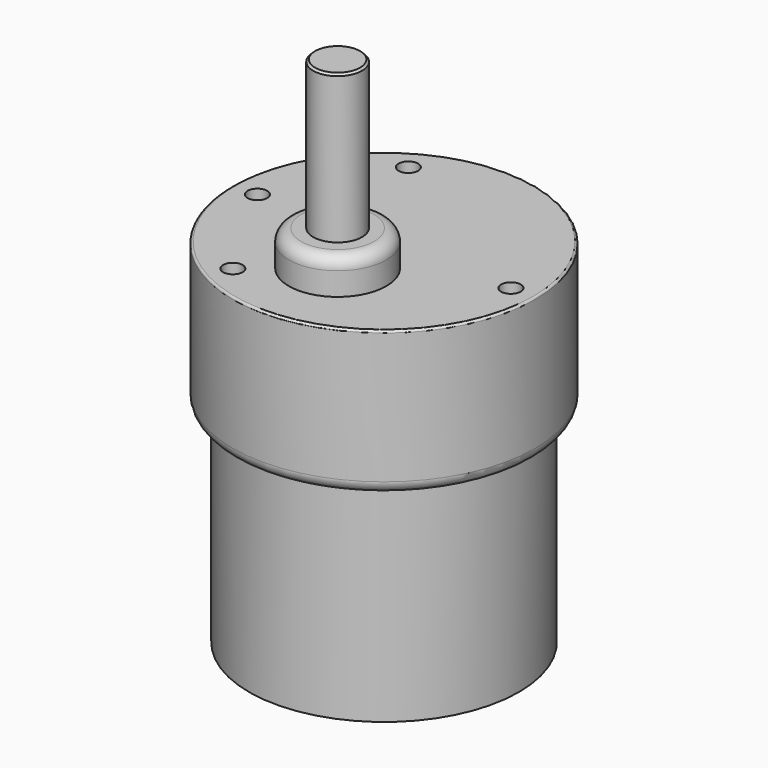
from build123d import *

# Parameters (mm, degrees)
F0_R         = 18.5
F0_R_2       = 16.51
F1_DEPTH     = 17.78
F2_R         = 5.969
F3_DEPTH     = 4.318
F4_R         = 3
F5_DEPTH     = 18.161
F7_DEPTH     = 12
F8_DEPTH     = 25.4
F9_R         = 4.445
F10_DEPTH    = 2.54
F11_R        = 0.635
F12_R        = 1.5
F13_R        = 1.5
F14_R        = 0.25
F15_T2_ANGLE = 276.1399558047
F15_T4_ANGLE = 96.0574088809
F16_D        = 2.4
F16_DEPTH    = 5
F16_TIP      = 0.7210327428


# Not quite as in the source:
# - a fillet or chamfer that OpenCascade refuses, or shapes differently, is made with other operations: its cross-section is extruded or revolved along the edge and cut away or added


with BuildPart() as f1:
    # F0 (on Top) → F1 (new body)
    with BuildSketch(Plane.XY):
        Circle(F0_R)
        Circle(F0_R_2, mode=Mode.SUBTRACT)
        Circle(F0_R_2)
    extrude(amount=F1_DEPTH)

    # F2 (on face) → F3 (join)
    with BuildSketch(Plane.XY.offset(17.78)):
        with Locations((0, -7.0954)):
            Circle(F2_R)
    extrude(amount=F3_DEPTH)

    # F0 (on Top) → F8 (join)
    with BuildSketch(Plane.XY):
        Circle(F0_R_2)
    extrude(amount=-F8_DEPTH)

    # F9 (on face) → F10 (join)
    with BuildSketch(Plane(origin=(0, 0, -25.4), x_dir=(1, 0, 0), z_dir=(0, 0, -1))):
        Circle(F9_R)
    extrude(amount=F10_DEPTH)

    # F11
    f11_edges = [f1.edges().sort_by_distance(p)[0] for p in [
        (-4.445, 0, -27.94),
    ]]
    fillet(f11_edges, radius=F11_R)

    # F12
    f12_edges = [f1.edges().sort_by_distance(p)[0] for p in [
        (-18.5, 0, 0),
    ]]
    fillet(f12_edges, radius=F12_R)

    # F13
    f13_edges = [f1.edges().sort_by_distance(p)[0] for p in [
        (-5.969, -7.0954, 22.098),
    ]]
    fillet(f13_edges, radius=F13_R)

    # F14
    f14_edges = [f1.edges().sort_by_distance(p)[0] for p in [
        (-18.5, 0, 17.78),
    ]]
    fillet(f14_edges, radius=F14_R)

    # F16
    with Locations(Plane.XY.offset(17.78)):
        with Locations((-7.7571209086, 13.4239), (-7.7571209086, -13.4239), (15.5039898493, 0.0177412977), (-15.5039898493, 0.0177412977)):
            Hole(F16_D / 2, depth=F16_DEPTH)
            with Locations((0, 0, -(F16_DEPTH + F16_TIP / 2))):  # 118° drill point
                Cone(0, F16_D / 2, F16_TIP, mode=Mode.SUBTRACT)


with BuildPart() as f5:
    # F4 (on face) → F5 (new body)
    with BuildSketch(Plane.XY.offset(22.098)):
        with Locations((0, -7.0954)):
            Circle(F4_R)
    extrude(amount=F5_DEPTH)

    # F6 (on face) → F7 (cut)
    with BuildSketch(Plane.XY.offset(40.259)):
        with BuildLine():
            ThreePointArc((1.1923271, -4.3425185847), (0, -4.0954), (-1.1923271, -4.3425185847))
            Line((-1.1923271, -4.3425185847), (1.1923271, -4.3425185847))
        make_face()
    extrude(amount=-F7_DEPTH, mode=Mode.SUBTRACT)

    # F15: chamfer of 0.25 on 2 edges, made by hand

    # F15_s1 → F15_t2 (revolve, cut)
    with BuildSketch(Plane(origin=(0.7545525529, -0.0811706499, 0), x_dir=(0, 0, 1), z_dir=(0.994263598, -0.1069574573, 0))):
        with BuildLine():
            Line((40.0019289322, 4.0476268655), (40.2660710678, 4.3117690011))
            Line((40.2660710678, 4.3117690011), (40.2710710678, 4.3117690011))
            ThreePointArc((40.2710710678, 4.3117690011), (40.264, 4.1832334672), (40.264, 4.0546979333))
            Line((40.264, 4.0546979333), (40.259, 4.0496979333))
            ThreePointArc((40.259, 4.0496979333), (40.1304644661, 4.0496979333), (40.0019289322, 4.0426268655))
            Line((40.0019289322, 4.0426268655), (40.0019289322, 4.0476268655))
        make_face()
    revolve(axis=Axis((0, -7.0954, 40.259), (0, 0, 1)), revolution_arc=F15_T2_ANGLE, mode=Mode.SUBTRACT)

    # F15_s3 → F15_t4 (revolve, cut)
    with BuildSketch(Plane.XZ.offset(7.0954)):
        with BuildLine():
            Line((3.0070710678, 40.0019289322), (2.7429289322, 40.2660710678))
            Line((2.7429289322, 40.2660710678), (2.7429289322, 40.2710710678))
            ThreePointArc((2.7429289322, 40.2710710678), (2.8714644661, 40.264), (3, 40.264))
            Line((3, 40.264), (3.005, 40.259))
            ThreePointArc((3.005, 40.259), (3.005, 40.1304644661), (3.0120710678, 40.0019289322))
            Line((3.0120710678, 40.0019289322), (3.0070710678, 40.0019289322))
        make_face()
    revolve(axis=Axis((0, -7.0954, 40.259), (0, 0, 1)), revolution_arc=F15_T4_ANGLE, mode=Mode.SUBTRACT)


solid = Compound([f1.part, f5.part])
